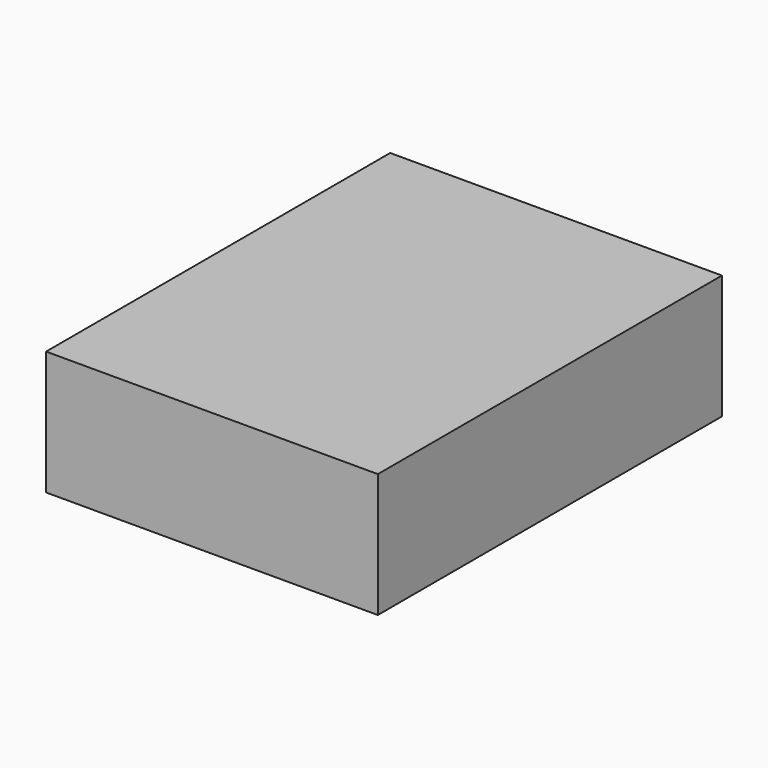
from build123d import *

# Parameters (mm, degrees)
F0_W     = 67.9279565811
F0_H     = 88.0647003651
F1_DEPTH = 25.4
F2_DEPTH = 25.4


# Not quite as in the source:
# - a feature of the source that left no trace in its solid (it failed there, or was rolled back) is left out


with BuildPart() as f1:
    # F0 (on Top) → F1 (new body)
    with BuildSketch(Plane.XY):
        Rectangle(F0_W, F0_H)
    extrude(amount=F1_DEPTH)


with BuildPart() as f2:
    # F0 (on Top) → F2 (new body)
    with BuildSketch(Plane.XY):
        Rectangle(F0_W, F0_H)
    extrude(amount=F2_DEPTH)


solid = Compound([f1.part, f2.part])
